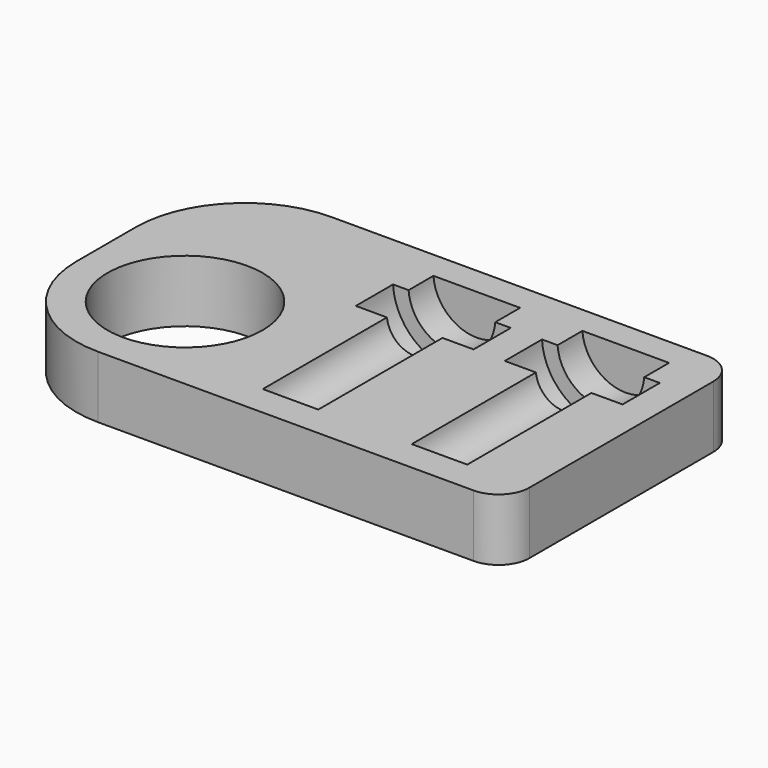
from build123d import *

# Parameters (mm, degrees)
F0_R         = 12.5
F1_DEPTH     = 10
F6_TEXT_SIZE = 5.5555555556
F7_DEPTH     = 1


# Not quite as in the source:
# - Text() gives the source's letters only with a copy of the font that has no kerning and outlines rounded to 1/6400 em; it was checked with that copy


with BuildPart() as f1:
    # F0 (on Top) → F1 (new body)
    with BuildSketch(Plane.XY):
        with BuildLine():
            ThreePointArc((0, 17.5), (5.1256313292, 5.1256313292), (17.5, 0))
            Line((17.5, 0), (78, 0))
            ThreePointArc((78, 0), (81.5355339059, 1.4644660941), (83, 5))
            Line((83, 5), (83, 42))
            ThreePointArc((83, 42), (81.5355339059, 45.5355339059), (78, 47))
            Line((78, 47), (17.5, 47))
            ThreePointArc((17.5, 47), (5.1256313292, 41.8743686708), (0, 29.5))
            Line((0, 29.5), (0, 17.5))
        make_face()
        with Locations((17.5, 17.5)):
            Circle(F0_R, mode=Mode.SUBTRACT)
    extrude(amount=F1_DEPTH)

    # F3 (on offset) → F4 (revolve, cut)
    with BuildSketch(Plane.XY.offset(10.5)):
        Polygon((44.5, 30), (44.5, 5), (49, 5), (49, 30), (54, 30), (54, 37.5), (51.5, 37.5), (51.5, 42.5), (44.5, 42.5), (44.5, 37.5), align=None)
    revolve(axis=Axis((44.5, 17.5, 10.5), (0, 1, 0)), mode=Mode.SUBTRACT)

    # F3 (on offset) → F5 (revolve, cut)
    with BuildSketch(Plane.XY.offset(10.5)):
        Polygon((68.5, 30), (68.5, 5), (73, 5), (73, 30), (78, 30), (78, 37.5), (75.5, 37.5), (75.5, 42.5), (68.5, 42.5), (68.5, 37.5), align=None)
    revolve(axis=Axis((68.5, 17.5, 10.5), (0, 1, 0)), mode=Mode.SUBTRACT)

    # F6 (on face) → F7 (cut)
    with BuildSketch(Plane(origin=(0, 0, 0), x_dir=(1, 0, 0), z_dir=(0, 0, -1))):
        with Locations((30, -9)):
            Text('821', F6_TEXT_SIZE, font='Open Sans', text_align=(TextAlign.LEFT, TextAlign.BOTTOM))
    extrude(amount=-F7_DEPTH, mode=Mode.SUBTRACT)


solid = f1.part
